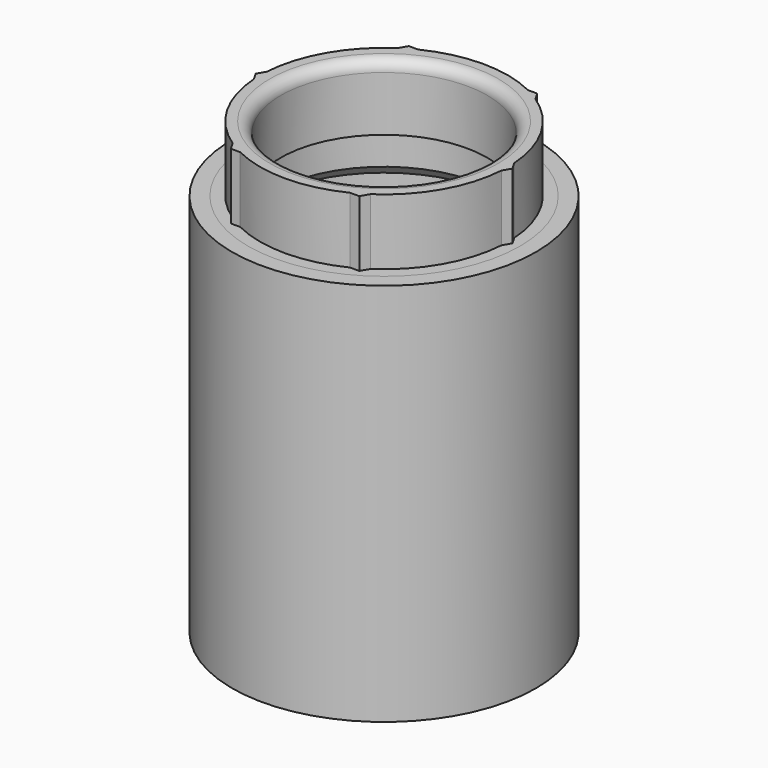
from build123d import *

# Parameters (mm, degrees)
F0_R     = 13.85
F0_R_2   = 11.7
F1_DEPTH = 35
F2_R     = 9.4254173389
F3_DEPTH = 6
F4_R     = 12.3979909048
F4_R_2   = 10.2650176462
F5_DEPTH = 4
F6_SIZE  = 1
F7_R     = 1
F8_R     = 12.25
F9_DEPTH = 7


with BuildPart() as f1:
    # F0 (on Top) → F1 (new body)
    with BuildSketch(Plane.XY):
        Circle(F0_R)
        Circle(F0_R_2, mode=Mode.SUBTRACT)
    extrude(amount=F1_DEPTH)

    # F8 (on face) → F9 (cut)
    with BuildSketch(Plane(origin=(0, 0, 0), x_dir=(1, 0, 0), z_dir=(0, 0, -1))):
        Circle(F8_R)
    extrude(amount=-F9_DEPTH, mode=Mode.SUBTRACT)


with BuildPart() as f3:
    # F2 (on face) → F3 (new body)
    with BuildSketch(Plane.XY.offset(35)):
        with BuildLine():
            ThreePointArc((11.276124747, -0.7341734743), (11.2940296095, -0.3672807911), (11.3, 0))
            ThreePointArc((11.3, 0), (11.2940296095, 0.3672807911), (11.276124747, 0.7341734743))
            Line((11.276124747, 0.7341734743), (6.273875253, 9.39832375))
            ThreePointArc((6.273875253, 9.39832375), (5.65, 9.7860870628), (5.002249494, 10.1324972243))
            Line((5.002249494, 10.1324972243), (-5.002249494, 10.1324972243))
            ThreePointArc((-5.002249494, 10.1324972243), (-5.65, 9.7860870628), (-6.273875253, 9.39832375))
            Line((-6.273875253, 9.39832375), (-11.276124747, 0.7341734743))
            ThreePointArc((-11.276124747, 0.7341734743), (-11.3, 0), (-11.276124747, -0.7341734743))
            Line((-11.276124747, -0.7341734743), (-6.273875253, -9.39832375))
            ThreePointArc((-6.273875253, -9.39832375), (-5.65, -9.7860870628), (-5.002249494, -10.1324972243))
            Line((-5.002249494, -10.1324972243), (5.002249494, -10.1324972243))
            ThreePointArc((5.002249494, -10.1324972243), (5.65, -9.7860870628), (6.273875253, -9.39832375))
            Line((6.273875253, -9.39832375), (11.276124747, -0.7341734743))
        make_face()
        Circle(F2_R, mode=Mode.SUBTRACT)
        with BuildLine():
            ThreePointArc((11.276124747, 0.7341734743), (11.2940296095, 0.3672807911), (11.3, 0))
            ThreePointArc((11.3, 0), (11.2940296095, -0.3672807911), (11.276124747, -0.7341734743))
            Line((11.276124747, -0.7341734743), (11.7, 0))
            Line((11.7, 0), (11.276124747, 0.7341734743))
        make_face()
        with BuildLine():
            Line((6.273875253, 9.39832375), (11.276124747, 0.7341734743))
            ThreePointArc((11.276124747, 0.7341734743), (9.7860870628, 5.65), (6.273875253, 9.39832375))
        make_face()
        with BuildLine():
            ThreePointArc((6.273875253, -9.39832375), (9.7860870628, -5.65), (11.276124747, -0.7341734743))
            Line((11.276124747, -0.7341734743), (6.273875253, -9.39832375))
        make_face()
        with BuildLine():
            ThreePointArc((5.002249494, 10.1324972243), (5.65, 9.7860870628), (6.273875253, 9.39832375))
            Line((6.273875253, 9.39832375), (5.85, 10.1324972243))
            Line((5.85, 10.1324972243), (5.002249494, 10.1324972243))
        make_face()
        with BuildLine():
            Line((5.85, -10.1324972243), (6.273875253, -9.39832375))
            ThreePointArc((6.273875253, -9.39832375), (5.65, -9.7860870628), (5.002249494, -10.1324972243))
            Line((5.002249494, -10.1324972243), (5.85, -10.1324972243))
        make_face()
        with BuildLine():
            Line((-5.002249494, 10.1324972243), (5.002249494, 10.1324972243))
            ThreePointArc((5.002249494, 10.1324972243), (0, 11.3), (-5.002249494, 10.1324972243))
        make_face()
        with BuildLine():
            ThreePointArc((-5.002249494, -10.1324972243), (0, -11.3), (5.002249494, -10.1324972243))
            Line((5.002249494, -10.1324972243), (-5.002249494, -10.1324972243))
        make_face()
        with BuildLine():
            ThreePointArc((-6.273875253, 9.39832375), (-5.65, 9.7860870628), (-5.002249494, 10.1324972243))
            Line((-5.002249494, 10.1324972243), (-5.85, 10.1324972243))
            Line((-5.85, 10.1324972243), (-6.273875253, 9.39832375))
        make_face()
        with BuildLine():
            Line((-5.85, -10.1324972243), (-5.002249494, -10.1324972243))
            ThreePointArc((-5.002249494, -10.1324972243), (-5.65, -9.7860870628), (-6.273875253, -9.39832375))
            Line((-6.273875253, -9.39832375), (-5.85, -10.1324972243))
        make_face()
        with BuildLine():
            Line((-11.276124747, 0.7341734743), (-6.273875253, 9.39832375))
            ThreePointArc((-6.273875253, 9.39832375), (-9.7860870628, 5.65), (-11.276124747, 0.7341734743))
        make_face()
        with BuildLine():
            ThreePointArc((-11.276124747, -0.7341734743), (-9.7860870628, -5.65), (-6.273875253, -9.39832375))
            Line((-6.273875253, -9.39832375), (-11.276124747, -0.7341734743))
        make_face()
        with BuildLine():
            ThreePointArc((-11.276124747, -0.7341734743), (-11.3, 0), (-11.276124747, 0.7341734743))
            Line((-11.276124747, 0.7341734743), (-11.7, 0))
            Line((-11.7, 0), (-11.276124747, -0.7341734743))
        make_face()
    extrude(amount=F3_DEPTH)

    # F4 (on face) → F5 (join)
    with BuildSketch(Plane.XY.offset(35)):
        Circle(F4_R)
        Circle(F4_R_2, mode=Mode.SUBTRACT)
    extrude(amount=-F5_DEPTH)

    # F6
    f6_edges = [f3.edges().sort_by_distance(p)[0] for p in [
        (-10.265018, 0, 31),
    ]]
    chamfer(f6_edges, length=F6_SIZE)

    # F7
    f7_edges = [f3.edges().sort_by_distance(p)[0] for p in [
        (-9.425417, 0, 41),
    ]]
    fillet(f7_edges, radius=F7_R)


solid = Compound([f1.part, f3.part])
